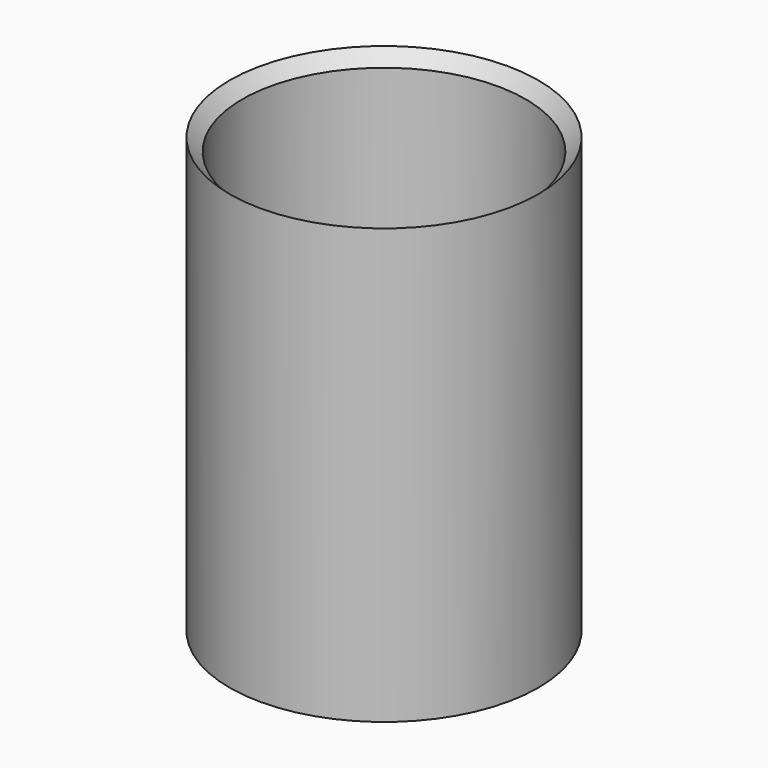
from build123d import *

# Parameters (mm, degrees)
F0_R     = 24.5
F1_DEPTH = 72
F2_T     = -2


# Not quite as in the source:
# - a fillet or chamfer that OpenCascade refuses, or shapes differently, is made with other operations: its cross-section is extruded or revolved along the edge and cut away or added


with BuildPart() as f1:
    # F0 (on Top) → F1 (new body)
    with BuildSketch(Plane.XY):
        Circle(F0_R)
    extrude(amount=F1_DEPTH)

    # F2
    f2_openings = [f1.faces().sort_by_distance(p)[0] for p in [
        (0, 0, 72),
    ]]
    offset(amount=F2_T, openings=f2_openings)

    # F3: chamfer of 5 on 1 edges, made by hand

    # F3_s1 → F3_t2 (revolve, cut)
    with BuildSketch(Plane.XZ):
        Polygon((27.5, 72), (22.5, 67), (22.5, 72), align=None)
    revolve(axis=Axis((0, 0, 72), (0, 0, 1)), mode=Mode.SUBTRACT)


solid = f1.part
